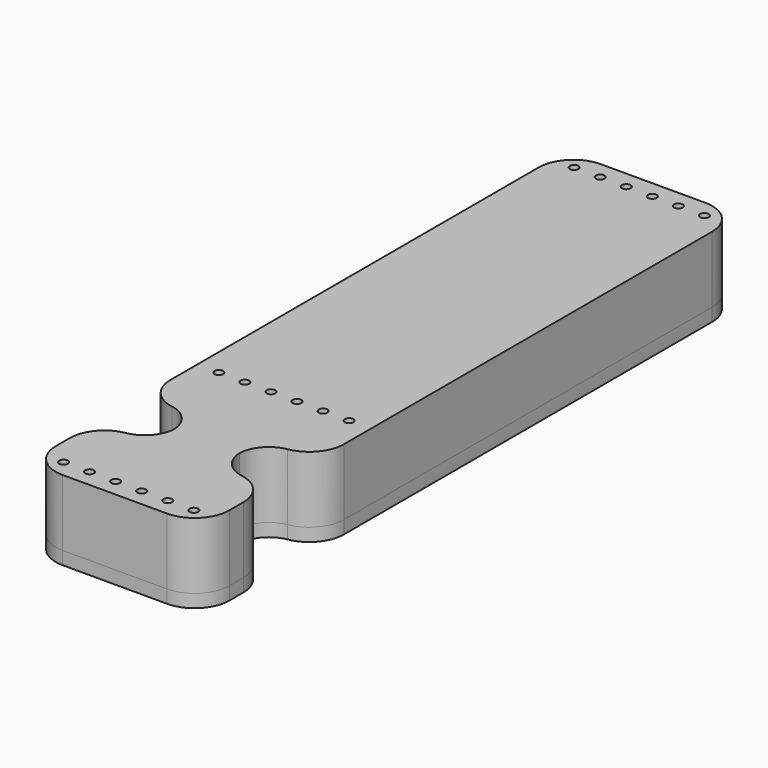
from build123d import *

# Parameters (mm, degrees)
F0_W        = 40
F0_H        = 155
F1_DEPTH    = 3
F2_W        = 12.5
F2_H        = 13
F3_DEPTH    = 3
F4_R        = 8
F5_T1_DEPTH = 3
F6_R        = 1
F7_DEPTH    = 3
F8_DEPTH    = 15.3


# Not quite as in the source:
# - a fillet or chamfer that OpenCascade refuses, or shapes differently, is made with other operations: its cross-section is extruded or revolved along the edge and cut away or added


with BuildPart() as f1:
    # F0 (on Top) → F1 (new body)
    with BuildSketch(Plane.XY):
        Rectangle(F0_W, F0_H)
    extrude(amount=F1_DEPTH)

    # F2 (on face) → F3 (cut, through all)
    with BuildSketch(Plane.XY.offset(3)):
        with Locations((-13.75, -51)):
            Rectangle(F2_W, F2_H)
        with Locations((13.75, -51)):
            Rectangle(F2_W, F2_H)
    extrude(amount=-F3_DEPTH, mode=Mode.SUBTRACT)

    # F4
    f4_edges = [f1.edges().sort_by_distance(p)[0] for p in [
        (-20, -44.5, 1.5),
        (20, -44.5, 1.5),
        (20, -57.5, 1.5),
        (-20, -57.5, 1.5),
        (-20, -77.5, 1.5),
        (20, -77.5, 1.5),
        (-20, 77.5, 1.5),
        (20, 77.5, 1.5),
    ]]
    fillet(f4_edges, radius=F4_R)

    # F5: fillet of radius 7 on 4 edges, made by hand

    # F5_s2 → F5_t1 (join)
    with BuildSketch(Plane.XY):
        with BuildLine():
            ThreePointArc((-13.3333333333, -44.3881063775), (-9.1536616892, -46.7717188872), (-7.5, -51.2901994578))
            Line((-7.5, -51.2901994578), (-6.8, -51.2901994578))
            Line((-6.8, -51.2901994578), (-6.8, -44.5))
            Line((-6.8, -44.5), (-7.5, -43.8))
            ThreePointArc((-7.5, -43.8), (-12, -43.8), (-13.2166666667, -43.6978970694))
            Line((-13.2166666667, -43.6978970694), (-13.3333333333, -44.3881063775))
        make_face()
        with BuildLine():
            ThreePointArc((-7.5, -50.7098005422), (-9.1536616892, -55.2282811128), (-13.3333333333, -57.6118936225))
            Line((-13.3333333333, -57.6118936225), (-13.2166666667, -58.3021029306))
            ThreePointArc((-13.2166666667, -58.3021029306), (-12, -58.2), (-7.5, -58.2))
            Line((-7.5, -58.2), (-6.8, -57.5))
            Line((-6.8, -57.5), (-6.8, -50.7098005422))
            Line((-6.8, -50.7098005422), (-7.5, -50.7098005422))
        make_face()
        with BuildLine():
            ThreePointArc((13.3333333333, -44.3881063775), (9.1536616892, -46.7717188872), (7.5, -51.2901994578))
            Line((7.5, -51.2901994578), (6.8, -51.2901994578))
            Line((6.8, -51.2901994578), (6.8, -44.5))
            Line((6.8, -44.5), (7.5, -43.8))
            ThreePointArc((7.5, -43.8), (12, -43.8), (13.2166666667, -43.6978970694))
            Line((13.2166666667, -43.6978970694), (13.3333333333, -44.3881063775))
        make_face()
        with BuildLine():
            ThreePointArc((7.5, -50.7098005422), (9.1536616892, -55.2282811128), (13.3333333333, -57.6118936225))
            Line((13.3333333333, -57.6118936225), (13.2166666667, -58.3021029306))
            ThreePointArc((13.2166666667, -58.3021029306), (12, -58.2), (7.5, -58.2))
            Line((7.5, -58.2), (6.8, -57.5))
            Line((6.8, -57.5), (6.8, -50.7098005422))
            Line((6.8, -50.7098005422), (7.5, -50.7098005422))
        make_face()
    extrude(amount=F5_T1_DEPTH)

    # F6 (on face) → F7 (cut, through all)
    with BuildSketch(Plane.XY.offset(3)):
        with Locations((-15, -73.5)):
            Circle(F6_R)
        with Locations((-9, -73.5)):
            Circle(F6_R)
        with Locations((-3, -73.5)):
            Circle(F6_R)
        with Locations((3, -73.5)):
            Circle(F6_R)
        with Locations((-15, -28.8)):
            Circle(F6_R)
        with Locations((-9, -28.8)):
            Circle(F6_R)
        with Locations((-3, -28.8)):
            Circle(F6_R)
        with Locations((3, -28.8)):
            Circle(F6_R)
        with Locations((-15, 73.5)):
            Circle(F6_R)
        with Locations((-9, 73.5)):
            Circle(F6_R)
        with Locations((-3, 73.5)):
            Circle(F6_R)
        with Locations((3, 73.5)):
            Circle(F6_R)
        with Locations((9, -73.5)):
            Circle(F6_R)
        with Locations((15, -73.5)):
            Circle(F6_R)
        with Locations((9, -28.8)):
            Circle(F6_R)
        with Locations((15, -28.8)):
            Circle(F6_R)
        with Locations((9, 73.5)):
            Circle(F6_R)
        with Locations((15, 73.5)):
            Circle(F6_R)
    extrude(amount=-F7_DEPTH, mode=Mode.SUBTRACT)

    # F8 (add): a face of the model
    f8_faces = [f1.faces().sort_by_distance(p)[0] for p in [
        (0, 3.1365524685, 3),
    ]]
    extrude(f8_faces, amount=F8_DEPTH)


solid = f1.part
